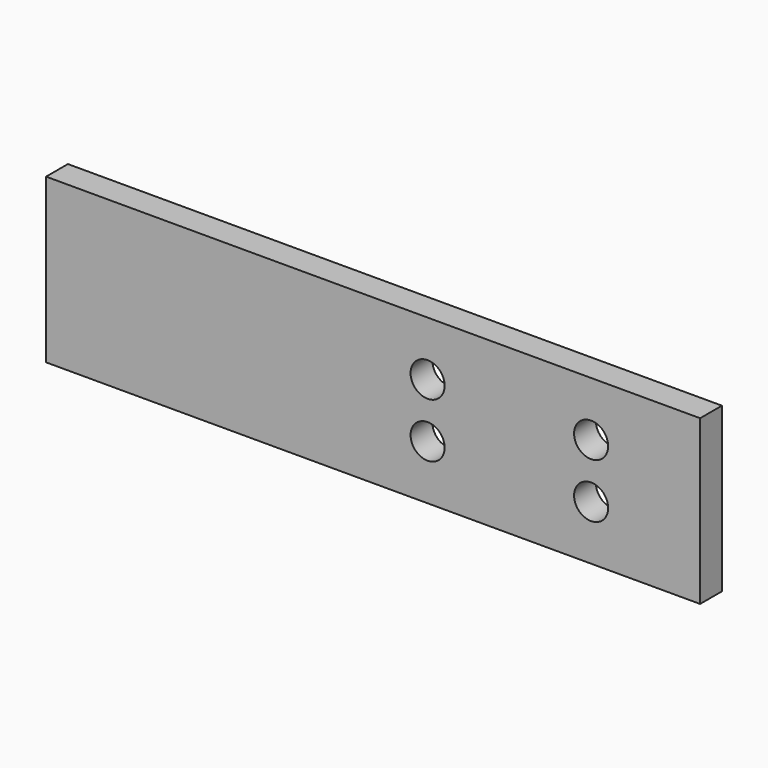
from build123d import *

# Parameters (mm, degrees)
F0_W     = 76.2
F0_H     = 19.05
F1_DEPTH = 1.5875
F4_R     = 1.984375
F2_R     = 1.984375
F3_R     = 1.984375
F5_R     = 1.984375
F6_DEPTH = 3.175


# Not quite as in the source:
# - a length typed as a fraction of an inch, garbled in the dataset ("3 / 203.2 mm" for 3/8 in), is restored


with BuildPart() as f1:
    # F0 (on Front) → F1 (new body, symmetric)
    with BuildSketch(Plane.XZ):
        Rectangle(F0_W, F0_H)
    extrude(amount=F1_DEPTH, both=True)

    # F4 (on face) + F2 (on face) + F3 (on face) + F5 (on face) → F6 (cut, through all)
    with BuildSketch(Plane.XZ.offset(1.5875)):
        with Locations((6.35, -3.175)):
            Circle(F4_R)
    with BuildSketch(Plane.XZ.offset(1.5875)):
        with Locations((25.4, 3.175)):
            Circle(F2_R)
    with BuildSketch(Plane.XZ.offset(1.5875)):
        with Locations((25.4, -3.175)):
            Circle(F3_R)
    with BuildSketch(Plane.XZ.offset(1.5875)):
        with Locations((6.35, 3.175)):
            Circle(F5_R)
    extrude(amount=-F6_DEPTH, mode=Mode.SUBTRACT)


solid = f1.part
